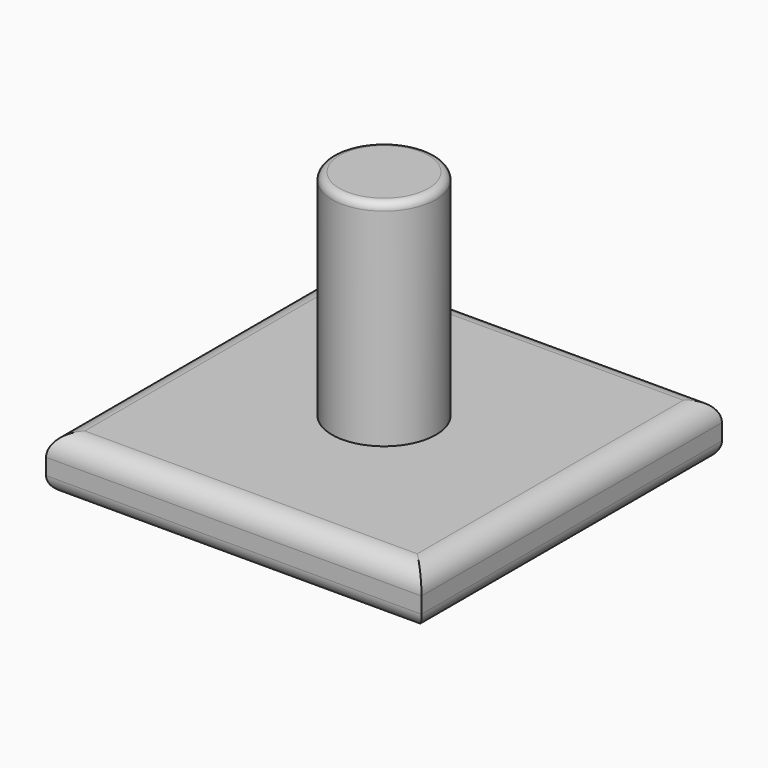
from build123d import *

# Parameters (mm, degrees)
F0_W     = 35
F0_H     = 35
F1_DEPTH = 5
F3_R     = 2
F4_R     = 1.5
F2_R     = 4.85
F5_DEPTH = 20
F6_R     = 0.7


with BuildPart() as f1:
    # F0 (on Top) → F1 (new body)
    with BuildSketch(Plane.XY):
        Rectangle(F0_W, F0_H)
    extrude(amount=-F1_DEPTH)

    # F3
    f3_edges = [f1.edges().sort_by_distance(p)[0] for p in [
        (0, -17.5, 0),
        (-17.5, 0, 0),
        (0, 17.5, 0),
        (17.5, 0, 0),
    ]]
    fillet(f3_edges, radius=F3_R)

    # F4
    f4_edges = [f1.edges().sort_by_distance(p)[0] for p in [
        (0, 17.5, -5),
        (-17.5, 0, -5),
        (0, -17.5, -5),
        (17.5, 0, -5),
    ]]
    fillet(f4_edges, radius=F4_R)

    # F2 (on Top) → F5 (join)
    with BuildSketch(Plane.XY):
        Circle(F2_R)
    extrude(amount=F5_DEPTH)

    # F6
    f6_edges = [f1.edges().sort_by_distance(p)[0] for p in [
        (-4.85, 0, 20),
    ]]
    fillet(f6_edges, radius=F6_R)


solid = f1.part
